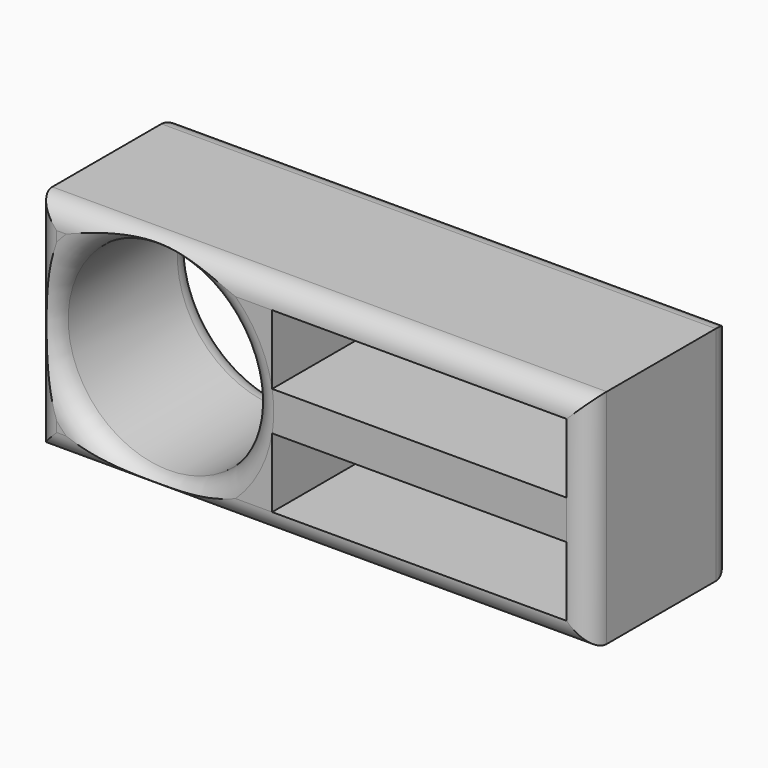
from build123d import *

# Parameters (mm, degrees)
F0_W        = 126.7489343882
F0_H        = 41.312854737
F1_DEPTH    = 25.4
F2_R        = 22.987
F3_DEPTH    = 41.313854737
F4_T1_DEPTH = 76.2
F4_T3_DEPTH = 152.1489343882
F5_T1_DEPTH = 152.1484343931
F5_T3_DEPTH = 76.1995000049
F6_W        = 67.343034428
F6_H        = 15.8471396435
F7_DEPTH    = 41.313854837


# Not quite as in the source:
# - a fillet or chamfer that OpenCascade refuses, or shapes differently, is made with other operations: its cross-section is extruded or revolved along the edge and cut away or added


with BuildPart() as f1:
    # F0 (on Top) → F1 (new body, symmetric)
    with BuildSketch(Plane.XY):
        Rectangle(F0_W, F0_H)
    extrude(amount=F1_DEPTH, both=True)

    # F2 (on face) → F3 (cut, through all)
    with BuildSketch(Plane.XZ.offset(20.6564273685)):
        with Locations((-36.7568694055, 0)):
            Circle(F2_R)
    extrude(amount=-F3_DEPTH, mode=Mode.SUBTRACT)

    # F4: fillet of radius 5.08 on 5 edges, made by hand

    # F4_s2 → F4_t1 (cut)
    with BuildSketch(Plane.XY.offset(-38.1)):
        with BuildLine():
            ThreePointArc((-63.3744671941, -15.5764273685), (-61.8865696425, -19.1685298169), (-58.2944671941, -20.6564273685))
            Line((-58.2944671941, -20.6564273685), (-63.3744671941, -20.6564273685))
            Line((-63.3744671941, -20.6564273685), (-63.3744671941, -15.5764273685))
        make_face()
        with BuildLine():
            ThreePointArc((63.3744671941, -15.5764273685), (61.8865696425, -19.1685298169), (58.2944671941, -20.6564273685))
            Line((58.2944671941, -20.6564273685), (63.3744671941, -20.6564273685))
            Line((63.3744671941, -20.6564273685), (63.3744671941, -15.5764273685))
        make_face()
    extrude(amount=F4_T1_DEPTH, mode=Mode.SUBTRACT)

    # F4_s4 → F4_t3 (cut)
    with BuildSketch(Plane.YZ.offset(-76.0744671941)):
        with BuildLine():
            ThreePointArc((-15.5764273685, -25.4), (-19.1685298169, -23.9121024484), (-20.6564273685, -20.32))
            Line((-20.6564273685, -20.32), (-20.6564273685, -25.4))
            Line((-20.6564273685, -25.4), (-15.5764273685, -25.4))
        make_face()
        with BuildLine():
            ThreePointArc((-15.5764273685, 25.4), (-19.1685298169, 23.9121024484), (-20.6564273685, 20.32))
            Line((-20.6564273685, 20.32), (-20.6564273685, 25.4))
            Line((-20.6564273685, 25.4), (-15.5764273685, 25.4))
        make_face()
    extrude(amount=F4_T3_DEPTH, mode=Mode.SUBTRACT)

    # F4_s5 → F4_t6 (revolve, cut)
    with BuildSketch(Plane.XY):
        with BuildLine():
            ThreePointArc((-13.7698694055, -15.5764273685), (-12.2819718539, -19.1685298169), (-8.6898694055, -20.6564273685))
            Line((-8.6898694055, -20.6564273685), (-13.7698694055, -20.6564273685))
            Line((-13.7698694055, -20.6564273685), (-13.7698694055, -15.5764273685))
        make_face()
    revolve(axis=Axis((-36.7568694055, -20.6564273685, 0), (0, -1, 0)), mode=Mode.SUBTRACT)

    # F5: fillet of radius 5.08 on 5 edges, made by hand

    # F5_s2 → F5_t1 (cut)
    with BuildSketch(Plane.YZ.offset(-76.0742171965)):
        with BuildLine():
            ThreePointArc((20.6565273685, -20.3201), (19.1686298169, -23.9122024484), (15.5765273685, -25.4001))
            Line((15.5765273685, -25.4001), (15.5765273685, -25.5017))
            ThreePointArc((15.5765273685, -25.5017), (18.1164773685, -25.5016), (20.6564273685, -25.5016))
            Line((20.6564273685, -25.5016), (20.7580273685, -25.4))
            ThreePointArc((20.7580273685, -25.4), (20.7580273685, -22.86005), (20.7581273685, -20.3201))
            Line((20.7581273685, -20.3201), (20.6565273685, -20.3201))
        make_face()
        with BuildLine():
            ThreePointArc((20.6565273685, 20.3201), (19.1686298169, 23.9122024484), (15.5765273685, 25.4001))
            Line((15.5765273685, 25.4001), (15.5765273685, 25.5017))
            ThreePointArc((15.5765273685, 25.5017), (18.1164773685, 25.5016), (20.6564273685, 25.5016))
            Line((20.6564273685, 25.5016), (20.7580273685, 25.4))
            ThreePointArc((20.7580273685, 25.4), (20.7580273685, 22.86005), (20.7581273685, 20.3201))
            Line((20.7581273685, 20.3201), (20.6565273685, 20.3201))
        make_face()
    extrude(amount=F5_T1_DEPTH, mode=Mode.SUBTRACT)

    # F5_s4 → F5_t3 (cut)
    with BuildSketch(Plane.XY.offset(-38.0997500025)):
        with BuildLine():
            ThreePointArc((58.2945671941, 20.6565273685), (61.8866696425, 19.1686298169), (63.3745671941, 15.5765273685))
            Line((63.3745671941, 15.5765273685), (63.4761671941, 15.5765273685))
            ThreePointArc((63.4761671941, 15.5765273685), (63.4760671941, 18.1164773685), (63.4760671941, 20.6564273685))
            Line((63.4760671941, 20.6564273685), (63.3744671941, 20.7580273685))
            ThreePointArc((63.3744671941, 20.7580273685), (60.8345171941, 20.7580273685), (58.2945671941, 20.7581273685))
            Line((58.2945671941, 20.7581273685), (58.2945671941, 20.6565273685))
        make_face()
        with BuildLine():
            ThreePointArc((-58.2945671941, 20.6565273685), (-61.8866696425, 19.1686298169), (-63.3745671941, 15.5765273685))
            Line((-63.3745671941, 15.5765273685), (-63.4761671941, 15.5765273685))
            ThreePointArc((-63.4761671941, 15.5765273685), (-63.4760671941, 18.1164773685), (-63.4760671941, 20.6564273685))
            Line((-63.4760671941, 20.6564273685), (-63.3744671941, 20.7580273685))
            ThreePointArc((-63.3744671941, 20.7580273685), (-60.8345171941, 20.7580273685), (-58.2945671941, 20.7581273685))
            Line((-58.2945671941, 20.7581273685), (-58.2945671941, 20.6565273685))
        make_face()
    extrude(amount=F5_T3_DEPTH, mode=Mode.SUBTRACT)

    # F5_s5 → F5_t6 (revolve, cut)
    with BuildSketch(Plane.XY):
        with BuildLine():
            ThreePointArc((-8.6899694055, 20.6565273685), (-12.2820718539, 19.1686298169), (-13.7699694055, 15.5765273685))
            Line((-13.7699694055, 15.5765273685), (-13.8715694055, 15.5765273685))
            ThreePointArc((-13.8715694055, 15.5765273685), (-13.8714694055, 18.1164773685), (-13.8714694055, 20.6564273685))
            Line((-13.8714694055, 20.6564273685), (-13.7698694055, 20.7580273685))
            ThreePointArc((-13.7698694055, 20.7580273685), (-11.2299194055, 20.7580273685), (-8.6899694055, 20.7581273685))
            Line((-8.6899694055, 20.7581273685), (-8.6899694055, 20.6565273685))
        make_face()
    revolve(axis=Axis((-36.7568694055, 20.6564273685, 0), (0, -1, 0)), mode=Mode.SUBTRACT)

    # F6 (on face) → F7 (cut, through all)
    with BuildSketch(Plane(origin=(0, 20.6564273685, 0), x_dir=(-1, 0, 0), z_dir=(0, 1, 0))):
        with Locations((-24.6229499801, -12.3964301783)):
            Rectangle(F6_W, F6_H)
        with Locations((-24.6229499801, 12.3964301783)):
            Rectangle(F6_W, F6_H)
    extrude(amount=-F7_DEPTH, mode=Mode.SUBTRACT)


solid = f1.part
